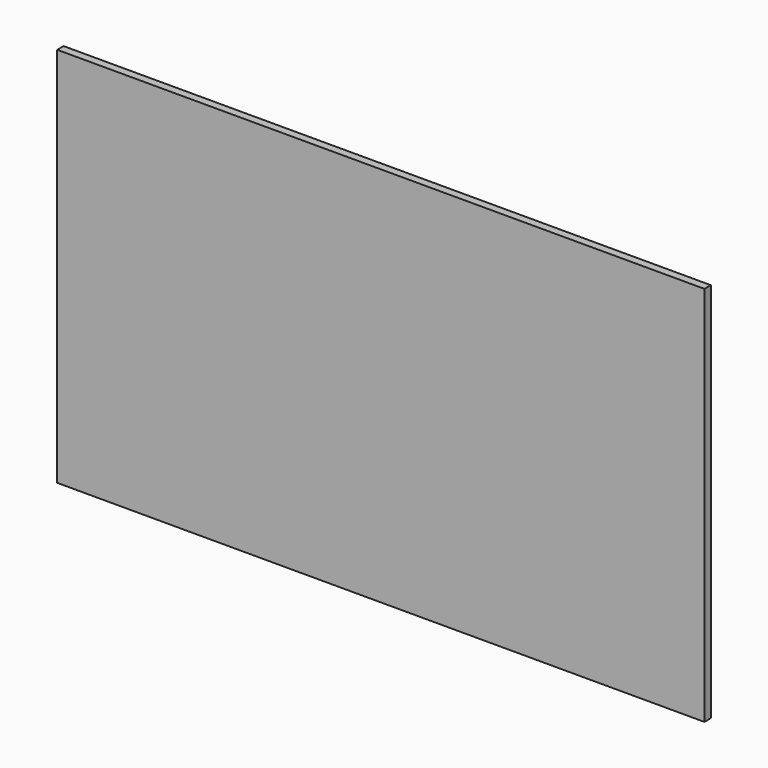
from build123d import *

# Parameters (mm, degrees)
F0_W     = 1282.7
F0_H     = 755.65
F1_DEPTH = 15.875


# Not quite as in the source:
# - a length typed as a fraction of an inch, garbled in the dataset ("3 / 203.2 mm" for 3/8 in), is restored


with BuildPart() as f1:
    # F0 (on Front) → F1 (new body)
    with BuildSketch(Plane.XZ):
        with Locations((641.35, 377.825)):
            Rectangle(F0_W, F0_H)
    extrude(amount=F1_DEPTH)


solid = f1.part
